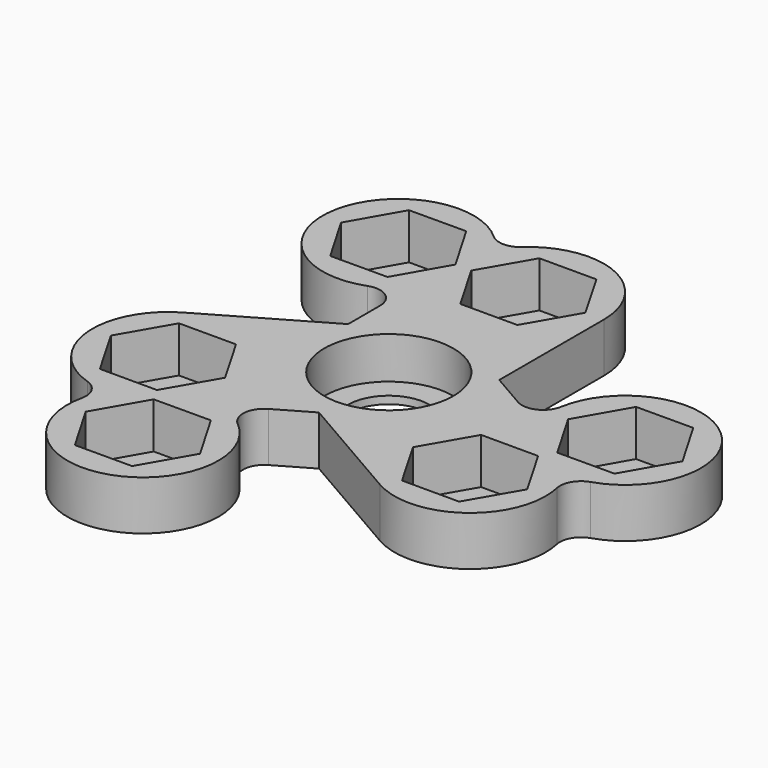
from build123d import *

# Parameters (mm, degrees)
F0_R     = 11.1
F0_R_2   = 7
F1_DEPTH = 8.5
F2_DEPTH = 7.9
F3_DEPTH = 7.2
F4_COUNT = 3
F5_R     = 3.6339158304


# Not quite as in the source:
# - a feature names something its author has since deleted; it is built from what else it names


with BuildPart() as f1:
    # F0 (on Top) → F1 (new body)
    with BuildSketch(Plane.XY):
        with BuildLine():
            ThreePointArc((-11.1881680787, 23.3799626101), (3.4317499164, 17.4611367137), (13, 30))
            ThreePointArc((13, 30), (3.4317499164, 42.5388632863), (-11.1881680787, 36.6200373899))
            ThreePointArc((-11.1881680787, 36.6200373899), (-35.2898051844, 31.4974370391), (-13, 20.9953167593))
            ThreePointArc((-13, 20.9953167593), (-12.0251844061, 22.1352903789), (-11.1881680787, 23.3799626101))
        make_face()
        Polygon((-17.4962580338, 38.5157601447), (-12.5614324777, 30.0316084449), (-17.4415106013, 21.5158483002), (-27.2564142809, 21.4842398553), (-32.1912398369, 29.9683915551), (-27.3111617133, 38.4841516998), align=None, mode=Mode.SUBTRACT)
        Polygon((4.9074772881, 38.5), (9.8149545762, 30), (4.9074772881, 21.5), (-4.9074772881, 21.5), (-9.8149545762, 30), (-4.9074772881, 38.5), align=None, mode=Mode.SUBTRACT)
        with BuildLine():
            ThreePointArc((-13, 0), (0, -13), (13, 0))
            ThreePointArc((13, 0), (0, 13), (-13, 0))
        make_face()
        Circle(F0_R, mode=Mode.SUBTRACT)
        Circle(F0_R)
        Circle(F0_R_2, mode=Mode.SUBTRACT)
        Polygon((4.9074772881, 21.5), (9.8149545762, 30), (4.9074772881, 38.5), (-4.9074772881, 38.5), (-9.8149545762, 30), (-4.9074772881, 21.5), align=None)
        Polygon((-17.4415106013, 21.5158483002), (-12.5614324777, 30.0316084449), (-17.4962580338, 38.5157601447), (-27.3111617133, 38.4841516998), (-32.1912398369, 29.9683915551), (-27.2564142809, 21.4842398553), align=None)
        with BuildLine():
            ThreePointArc((-13, 0), (0, 13), (13, 0))
            Line((13, 0), (13, 30))
            ThreePointArc((13, 30), (3.4317499164, 17.4611367137), (-11.1881680787, 23.3799626101))
            ThreePointArc((-11.1881680787, 23.3799626101), (-12.0251844061, 22.1352903789), (-13, 20.9953167593))
            Line((-13, 20.9953167593), (-13, 0))
        make_face()
    extrude(amount=-F1_DEPTH)

    # F0 (on Top) → F2 (cut)
    with BuildSketch(Plane.XY):
        Polygon((4.9074772881, 21.5), (9.8149545762, 30), (4.9074772881, 38.5), (-4.9074772881, 38.5), (-9.8149545762, 30), (-4.9074772881, 21.5), align=None)
        Polygon((-17.4415106013, 21.5158483002), (-12.5614324777, 30.0316084449), (-17.4962580338, 38.5157601447), (-27.3111617133, 38.4841516998), (-32.1912398369, 29.9683915551), (-27.2564142809, 21.4842398553), align=None)
    extrude(amount=-F2_DEPTH, mode=Mode.SUBTRACT)

    # F0 (on Top) → F3 (cut)
    with BuildSketch(Plane.XY):
        Circle(F0_R)
        Circle(F0_R_2, mode=Mode.SUBTRACT)
    extrude(amount=-F3_DEPTH, mode=Mode.SUBTRACT)

    # F4: F1 ×3 about axis
    f4_axis = Axis((0, 0, 0), (0, 0, 1))


with BuildPart() as f1_1:
    add(f1.part)
    for i in range(1, F4_COUNT):
        add(f1.part.rotate(f4_axis, i * 360 / F4_COUNT))

    # F5
    f5_edges = [f1_1.edges().sort_by_distance(p)[0] for p in [
        (-13, 20.995317, -4.25),
        (-11.188168, 36.620037, -4.25),
        (-11.682478, -21.755989, -4.25),
        (-26.119799, -27.999256, -4.25),
        (37.307967, -8.620781, -4.25),
        (24.682478, 0.760672, -4.25),
    ]]
    fillet(f5_edges, radius=F5_R)


solid = f1_1.part
